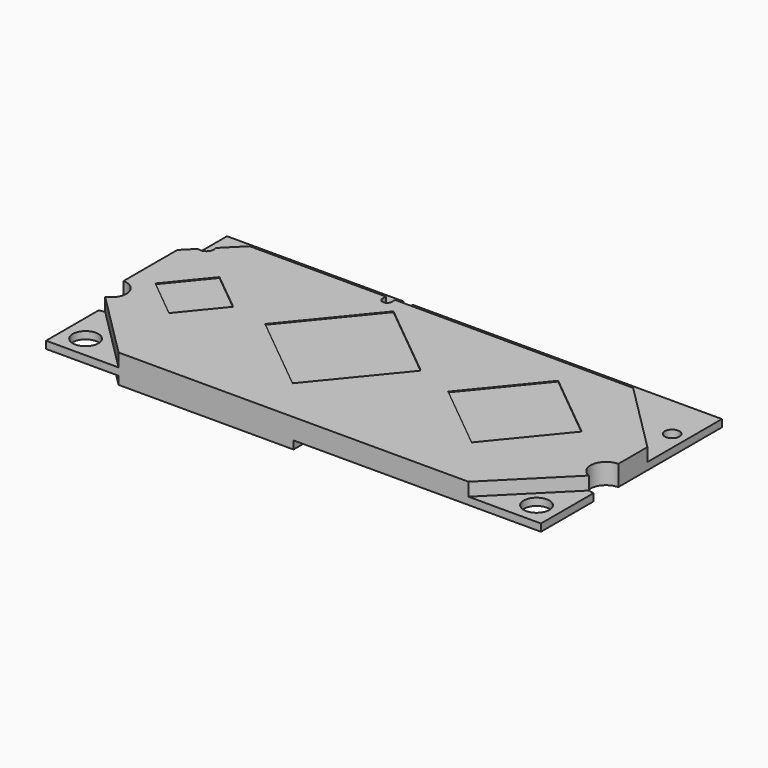
from build123d import *
from build123d import SkipClean  # not in build123d's __all__

# Parameters (mm, degrees)
F0_W     = 8.45
F0_H     = 3
F0_R     = 1.75
F0_R_2   = 1
F1_DEPTH = 1
F2_DEPTH = 2.1
F3_DEPTH = 1.8
F5_START = 1.7
F5_DEPTH = 0.3


with BuildPart() as f1:
    # F0 (on Top) → F1 (new body)
    with BuildSketch(Plane.XY):
        with Locations((29.575, -1.5)):
            Rectangle(F0_W, F0_H)
        Polygon((33.8, 0), (33.8, -3), (57.8720779386, -3), (54.8720779386, 0), align=None)
        Polygon((54.8720779386, 0), (57.8720779386, -3), (67.6, -3), (67.6, 0), align=None)
        with BuildLine():
            Line((66.8420563389, -21.7584487245), (57.7005050634, -30.9))
            Line((57.7005050634, -30.9), (67.6, -30.9))
            Line((67.6, -30.9), (67.6, -21.9))
            ThreePointArc((67.6, -21.9), (67.2144758902, -21.8643088821), (66.8420563389, -21.7584487245))
        make_face()
        with Locations((64.6, -27.9)):
            Circle(F0_R, mode=Mode.SUBTRACT)
        with BuildLine():
            Line((33.8, -3), (33.8, -30.9))
            Line((33.8, -30.9), (57.7005050634, -30.9))
            Line((57.7005050634, -30.9), (66.8420563389, -21.7584487245))
            ThreePointArc((66.8420563389, -21.7584487245), (65.5356911179, -19.4144758902), (67.6, -17.7))
            Line((67.6, -17.7), (67.6, -12.7279220614))
            Line((67.6, -12.7279220614), (57.8720779386, -3))
            Line((57.8720779386, -3), (33.8, -3))
        make_face()
        with BuildLine():
            Line((24.1, -3), (5.4852813742, -3))
            Line((5.4852813742, -3), (2.9068134786, -5.5784678956))
            ThreePointArc((2.9068134786, -5.5784678956), (2.9764254909, -5.7841452787), (3, -6))
            ThreePointArc((3, -6), (2.5378047488, -6.8430694231), (1.5784678956, -6.9068134786))
            Line((1.5784678956, -6.9068134786), (0, -8.4852813742))
            Line((0, -8.4852813742), (0, -17.7))
            ThreePointArc((0, -17.7), (2.0643088821, -19.4144758902), (0.7579436611, -21.7584487245))
            Line((0.7579436611, -21.7584487245), (9.8994949366, -30.9))
            Line((9.8994949366, -30.9), (33.8, -30.9))
            Line((33.8, -30.9), (33.8, -3))
            Line((33.8, -3), (25.35, -3))
            Line((25.35, -3), (25.35, -3.575))
            ThreePointArc((25.35, -3.575), (24.725, -4.2), (24.1, -3.575))
            Line((24.1, -3.575), (24.1, -3))
        make_face()
        with BuildLine():
            Line((9.8994949366, -30.9), (0.7579436611, -21.7584487245))
            ThreePointArc((0.7579436611, -21.7584487245), (0.3855241098, -21.8643088821), (0, -21.9))
            Line((0, -21.9), (0, -30.9))
            Line((0, -30.9), (9.8994949366, -30.9))
        make_face()
        with Locations((3, -27.9)):
            Circle(F0_R, mode=Mode.SUBTRACT)
        Polygon((8.4852813742, 0), (0, 0), (0, -3), (5.4852813742, -3), align=None)
        Polygon((24.1, 0), (8.4852813742, 0), (5.4852813742, -3), (24.1, -3), align=None)
        with BuildLine():
            Line((5.4852813742, -3), (0, -3))
            Line((0, -3), (0, -8.4852813742))
            Line((0, -8.4852813742), (1.5784678956, -6.9068134786))
            ThreePointArc((1.5784678956, -6.9068134786), (1.2928932188, -5.2928932188), (2.9068134786, -5.5784678956))
            Line((2.9068134786, -5.5784678956), (5.4852813742, -3))
        make_face()
        Polygon((67.6, -3), (57.8720779386, -3), (67.6, -12.7279220614), align=None)
        with Locations((65.6, -6)):
            Circle(F0_R_2, mode=Mode.SUBTRACT)
    extrude(amount=-F1_DEPTH)

    # F0 (on Top) → F2 (join)
    with BuildSketch(Plane.XY):
        with BuildLine():
            Line((24.1, -3), (5.4852813742, -3))
            Line((5.4852813742, -3), (2.9068134786, -5.5784678956))
            ThreePointArc((2.9068134786, -5.5784678956), (2.9764254909, -5.7841452787), (3, -6))
            ThreePointArc((3, -6), (2.5378047488, -6.8430694231), (1.5784678956, -6.9068134786))
            Line((1.5784678956, -6.9068134786), (0, -8.4852813742))
            Line((0, -8.4852813742), (0, -17.7))
            ThreePointArc((0, -17.7), (2.0643088821, -19.4144758902), (0.7579436611, -21.7584487245))
            Line((0.7579436611, -21.7584487245), (9.8994949366, -30.9))
            Line((9.8994949366, -30.9), (33.8, -30.9))
            Line((33.8, -30.9), (33.8, -3))
            Line((33.8, -3), (25.35, -3))
            Line((25.35, -3), (25.35, -3.575))
            ThreePointArc((25.35, -3.575), (24.725, -4.2), (24.1, -3.575))
            Line((24.1, -3.575), (24.1, -3))
        make_face()
    with SkipClean():  # cleaning this boolean's faces spoils the solid; the shape is the same uncleaned
        extrude(amount=-F2_DEPTH)

    # F0 (on Top) → F3 (join)
    with BuildSketch(Plane.XY):
        with BuildLine():
            Line((24.1, -3), (5.4852813742, -3))
            Line((5.4852813742, -3), (2.9068134786, -5.5784678956))
            ThreePointArc((2.9068134786, -5.5784678956), (2.9764254909, -5.7841452787), (3, -6))
            ThreePointArc((3, -6), (2.5378047488, -6.8430694231), (1.5784678956, -6.9068134786))
            Line((1.5784678956, -6.9068134786), (0, -8.4852813742))
            Line((0, -8.4852813742), (0, -17.7))
            ThreePointArc((0, -17.7), (2.0643088821, -19.4144758902), (0.7579436611, -21.7584487245))
            Line((0.7579436611, -21.7584487245), (9.8994949366, -30.9))
            Line((9.8994949366, -30.9), (33.8, -30.9))
            Line((33.8, -30.9), (33.8, -3))
            Line((33.8, -3), (25.35, -3))
            Line((25.35, -3), (25.35, -3.575))
            ThreePointArc((25.35, -3.575), (24.725, -4.2), (24.1, -3.575))
            Line((24.1, -3.575), (24.1, -3))
        make_face()
        with BuildLine():
            Line((33.8, -3), (33.8, -30.9))
            Line((33.8, -30.9), (57.7005050634, -30.9))
            Line((57.7005050634, -30.9), (66.8420563389, -21.7584487245))
            ThreePointArc((66.8420563389, -21.7584487245), (65.5356911179, -19.4144758902), (67.6, -17.7))
            Line((67.6, -17.7), (67.6, -12.7279220614))
            Line((67.6, -12.7279220614), (57.8720779386, -3))
            Line((57.8720779386, -3), (33.8, -3))
        make_face()
    extrude(amount=F3_DEPTH)

    # F4 (on Top) → F5 (cut)
    with BuildSketch(Plane.XY.offset(F5_START)):
        Polygon((8.4177003427, -20.4326654506), (12.8503657933, -15.014965108), (7.4326654506, -10.5822996573), (3, -16), align=None)
        Polygon((37.7007315866, -14.0299302159), (26.8653309013, -5.1645993147), (18, -16), (28.8354006853, -24.8653309013), align=None)
        Polygon((52.2874863017, -23.5988550582), (59.8863413599, -14.3113687565), (50.5988550582, -6.7125136983), (43, -16), align=None)
    extrude(amount=F5_DEPTH, mode=Mode.SUBTRACT)


solid = f1.part
